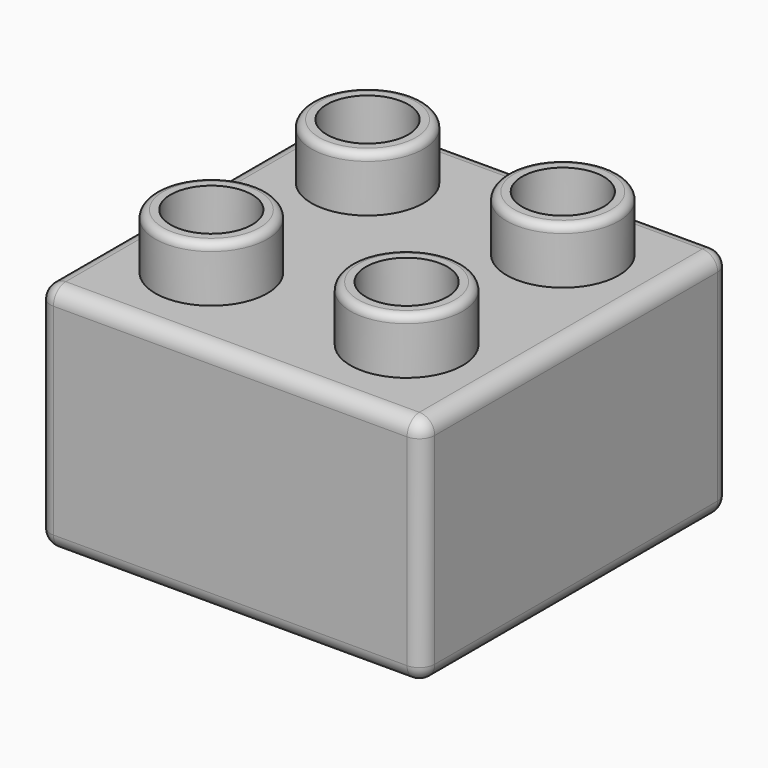
from build123d import *

# Parameters (mm, degrees)
F0_W          = 31.75
F0_H          = 31.75
F5_DEPTH      = 19.177
F1_W          = 28.575
F1_H          = 28.575
F6_DEPTH      = 18.161
F6_DEPTH_BACK = 0.381
F2_R          = 6.5405
F7_DEPTH      = 15.875
F3_R          = 5.461
F8_DEPTH      = 15.875
F8_DEPTH_BACK = 0.635
F4_W          = 1.016
F4_H          = 1.905
F10_DEPTH     = 17.526
F15_ANGLE     = 90
F16_R         = 4.6355
F18_DEPTH     = 4.699
F17_R         = 3.3655
F19_DEPTH     = 4.699
F23_R         = 1.26999
F24_R         = 0.635
F24_2_R       = 0.635
F24_3_R       = 0.635
F24_4_R       = 0.635


# Not quite as in the source:
# - a fillet or chamfer is up to 0.001 mm smaller than in the source, because OpenCascade refuses the exact size


with BuildPart() as f5:
    # F0 (on Top) → F5 (new body)
    with BuildSketch(Plane.XY):
        with Locations((0, -0.3175)):
            Rectangle(F0_W, F0_H)
    extrude(amount=F5_DEPTH)

    # F1 (on face) → F6 (cut, two sides)
    with BuildSketch(Plane.XY) as f6_sk:
        Rectangle(F1_W, F1_H)
    extrude(amount=F6_DEPTH, mode=Mode.SUBTRACT)
    extrude(f6_sk.sketch, amount=-F6_DEPTH_BACK, mode=Mode.SUBTRACT)

    # F23 (radius 1.27 in the source; OpenCascade refuses exactly that, so slightly less here)
    f23_edges = [f5.edges().sort_by_distance(p)[0] for p in [
        (0, -16.1925, 19.177),
        (-15.875, -0.3175, 19.177),
        (0, 15.5575, 19.177),
        (15.875, -0.3175, 19.177),
        (-15.875, -16.1925, 9.5885),
        (15.875, -16.1925, 9.5885),
        (-15.875, 15.5575, 9.5885),
        (15.875, 15.5575, 9.5885),
        (15.875, -0.3175, 0),
        (0, -16.1925, 0),
        (-15.875, -0.3175, 0),
        (0, 15.5575, 0),
    ]]
    fillet(f23_edges, radius=F23_R)


with BuildPart() as f7:
    # F2 (on face) → F7 (new body)
    with BuildSketch(Plane.XY):
        Circle(F2_R)
    extrude(amount=F7_DEPTH)

    # F3 (on face) → F8 (cut, two sides)
    with BuildSketch(Plane.XY) as f8_sk:
        Circle(F3_R)
    extrude(amount=F8_DEPTH, mode=Mode.SUBTRACT)
    extrude(f8_sk.sketch, amount=-F8_DEPTH_BACK, mode=Mode.SUBTRACT)


with BuildPart() as f7_1:
    # F9: moved
    add(f7.part.moved(Location((0, 0, 2.286))))


with BuildPart() as f10:
    # F4 (on face) → F10 (new body)
    with BuildSketch(Plane.XY):
        Rectangle(F4_W, F4_H)
    extrude(amount=F10_DEPTH)


with BuildPart() as f10_1:
    # F11: moved
    add(f10.part.moved(Location((8.0645, 13.8557, 0.635))))


with BuildPart() as f12_1:
    # F12: instance of F10
    add(f10_1.part.mirror(Plane.XZ))


with BuildPart() as f13_1:
    # F13: instance of F12_1
    add(f12_1.part.mirror(Plane.YZ))


with BuildPart() as f13_2:
    # F13: instance of F10
    add(f10_1.part.mirror(Plane.YZ))


with BuildPart() as f15_1:
    # F15: copy of F12_1
    add(f12_1.part.rotate(Axis((0, 0, 4.273429513), (0, 0, -1)), F15_ANGLE))


with BuildPart() as f15_2:
    # F15: copy of F13_1
    add(f13_1.part.rotate(Axis((0, 0, 4.273429513), (0, 0, -1)), F15_ANGLE))


with BuildPart() as f15_3:
    # F15: copy of F10
    add(f10_1.part.rotate(Axis((0, 0, 4.273429513), (0, 0, -1)), F15_ANGLE))


with BuildPart() as f15_4:
    # F15: copy of F13_2
    add(f13_2.part.rotate(Axis((0, 0, 4.273429513), (0, 0, -1)), F15_ANGLE))


with BuildPart() as f18:
    # F16 (on Top) → F18 (new body)
    with BuildSketch(Plane.XY):
        Circle(F16_R)
    extrude(amount=F18_DEPTH)

    # F17 (on Top) → F19 (cut)
    with BuildSketch(Plane.XY):
        Circle(F17_R)
    extrude(amount=F19_DEPTH, mode=Mode.SUBTRACT)


with BuildPart() as f18_1:
    # F20: moved
    add(f18.part.moved(Location((8.0645, 8.0645, 19.05))))


with BuildPart() as f21_1:
    # F21: instance of F18
    add(f18_1.part.mirror(Plane.XZ))


with BuildPart() as f22_1:
    # F22: instance of F18
    add(f18_1.part.mirror(Plane.YZ))

    # F24
    f24_edges = [f22_1.edges().sort_by_distance(p)[0] for p in [
        (-3.429, 8.0645, 23.749),
    ]]
    fillet(f24_edges, radius=F24_R)


with BuildPart() as f22_2:
    # F22: instance of F21_1
    add(f21_1.part.mirror(Plane.YZ))

    # F24#4
    f24_4_edges = [f22_2.edges().sort_by_distance(p)[0] for p in [
        (-3.429, -8.0645, 23.749),
    ]]
    fillet(f24_4_edges, radius=F24_4_R)


with BuildPart() as f18_2:
    add(f18_1.part)

    # F24#2
    f24_2_edges = [f18_2.edges().sort_by_distance(p)[0] for p in [
        (3.429, 8.0645, 23.749),
    ]]
    fillet(f24_2_edges, radius=F24_2_R)


with BuildPart() as f21_1_1:
    add(f21_1.part)

    # F24#3
    f24_3_edges = [f21_1_1.edges().sort_by_distance(p)[0] for p in [
        (3.429, -8.0645, 23.749),
    ]]
    fillet(f24_3_edges, radius=F24_3_R)


with BuildPart() as f15_3_1:
    add(f15_3.part)

    # F25: union F21_1, F5, F7, F12_1, F13_2, F13_1, F15_1, F15_4, F15_2, F18, F22_1, F22_2, F10
    add(f21_1_1.part)
    add(f5.part)
    add(f7_1.part)
    add(f12_1.part)
    add(f13_2.part)
    add(f13_1.part)
    add(f15_1.part)
    add(f15_4.part)
    add(f15_2.part)
    add(f18_2.part)
    add(f22_1.part)
    add(f22_2.part)
    add(f10_1.part)


solid = f15_3_1.part
